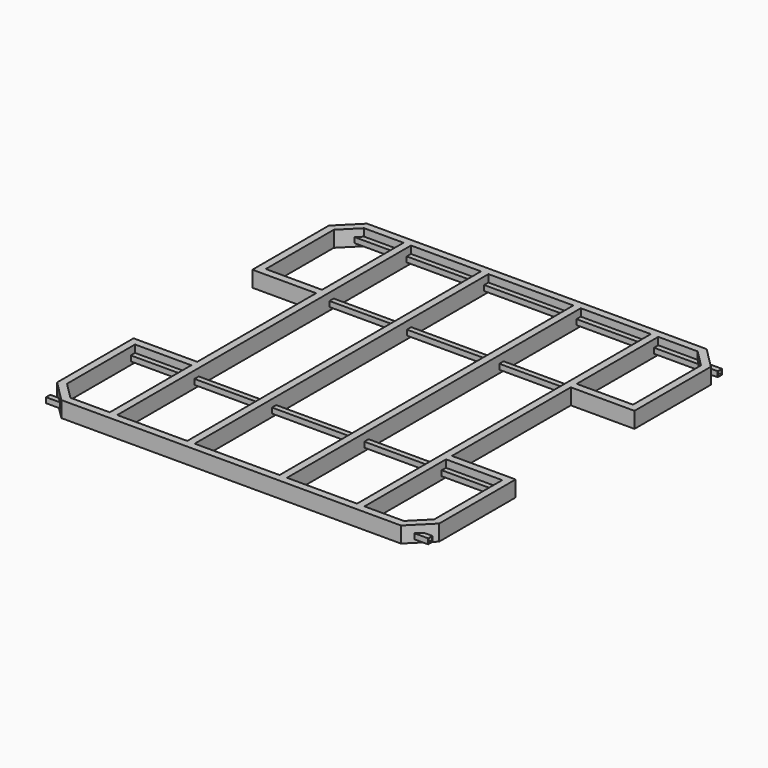
from build123d import *

# Parameters (mm, degrees)
F2_DEPTH = 75
F3_W     = 25
F3_H     = 25
F3_W_2   = 21.8
F3_H_2   = 21.8
F4_DEPTH = 1800


# Not quite as in the source:
# - the program builds the solid bodies; features that only make, move or delete a surface that nothing else refers to are left out


with BuildPart() as f2:
    # F1 (on face) → F2 (new body)
    with BuildSketch(Plane.XY):
        Polygon((-300, 1068.4480190277), (-300, 1768.4480190277), (0, 1768.4480190277), (0, 2218.4480190277), (-100, 2318.4480190277), (-1700, 2318.4480190277), (-1800, 2218.4480190277), (-1800, 1768.4480190277), (-1500, 1768.4480190277), (-1500, 1068.4480190277), (-1800, 1068.4480190277), (-1800, 618.4480190277), (-1700, 518.4480190277), (-100, 518.4480190277), (0, 618.4480190277), (0, 1068.4480190277), align=None)
        Polygon((-1500, 553.4480190277), (-1685.5025253169, 553.4480190277), (-1765, 632.9454937108), (-1765, 1033.4480190277), (-1500, 1033.4480190277), align=None, mode=Mode.SUBTRACT)
        Polygon((-300, 1033.4480190277), (-35, 1033.4480190277), (-35, 632.9454937108), (-114.4974746831, 553.4480190277), (-300, 553.4480190277), align=None, mode=Mode.SUBTRACT)
        Polygon((-1465, 1033.4480190277), (-1465, 1803.4480190277), (-1465, 2283.4480190277), (-1135, 2283.4480190277), (-1135, 553.4480190277), (-1465, 553.4480190277), align=None, mode=Mode.SUBTRACT)
        Polygon((-1765, 2203.9505443447), (-1685.5025253169, 2283.4480190277), (-1500, 2283.4480190277), (-1500, 1803.4480190277), (-1765, 1803.4480190277), align=None, mode=Mode.SUBTRACT)
        Polygon((-735, 553.4480190277), (-875, 553.4480190277), (-1100, 553.4480190277), (-1100, 2283.4480190277), (-875, 2283.4480190277), (-735, 2283.4480190277), (-700, 2283.4480190277), (-700, 553.4480190277), align=None, mode=Mode.SUBTRACT)
        Polygon((-335, 1803.4480190277), (-335, 1033.4480190277), (-335, 553.4480190277), (-665, 553.4480190277), (-665, 2283.4480190277), (-335, 2283.4480190277), align=None, mode=Mode.SUBTRACT)
        Polygon((-300, 2283.4480190277), (-114.4974746831, 2283.4480190277), (-35, 2203.9505443447), (-35, 1803.4480190277), (-300, 1803.4480190277), align=None, mode=Mode.SUBTRACT)
    extrude(amount=F2_DEPTH)

    # F3 (on face) → F4 (join)
    with BuildSketch(Plane(origin=(-1800, 0, 0), x_dir=(0, -1, 0), z_dir=(-1, 0, 0))):
        with Locations((-565.9480190277, 27.5)):
            Rectangle(F3_W, F3_H)
        with Locations((-565.9480190277, 27.5)):
            Rectangle(F3_W_2, F3_H_2, mode=Mode.SUBTRACT)
        with Locations((-1020.9480190277, 27.5)):
            Rectangle(F3_W, F3_H)
        with Locations((-1020.9480190277, 27.5)):
            Rectangle(F3_W_2, F3_H_2, mode=Mode.SUBTRACT)
    extrude(amount=-F4_DEPTH)

    # F7: F2 across plane


with BuildPart() as f2_1:
    add(f2.part)
    add(f2.part.mirror(Plane(origin=(-900, 1418.4480190277, 37.5), x_dir=(-1, 0, 0), z_dir=(0, 1, 0))))


solid = f2_1.part
